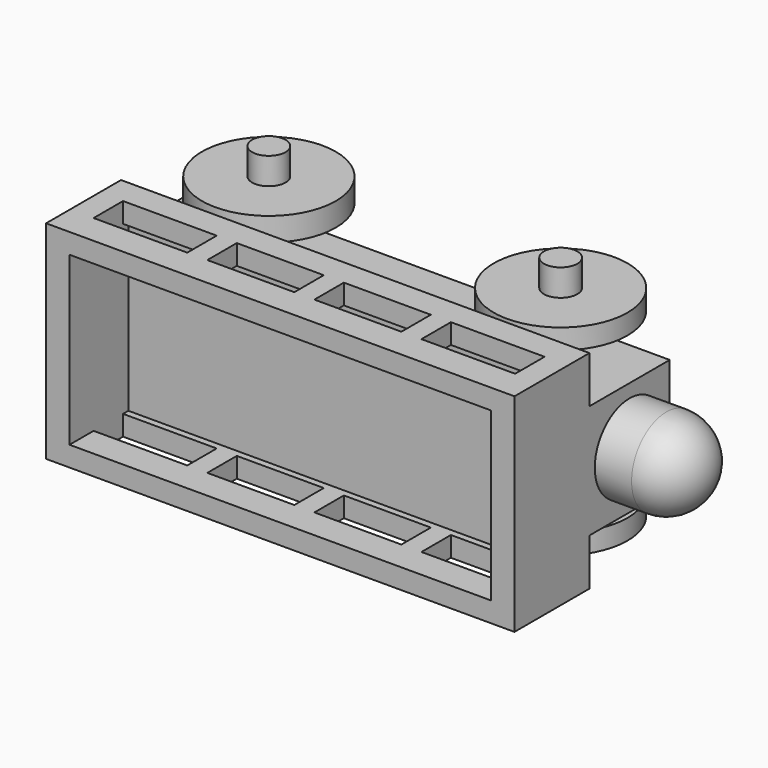
from build123d import *

# Parameters (mm, degrees)
F0_W      = 70
F0_H      = 31
F1_DEPTH  = 1.5
F2_W      = 70
F2_H      = 3
F3_DEPTH  = 11
F4_W      = 70
F4_H      = 3
F5_DEPTH  = 11
F6_W      = 3.5
F6_H      = 25
F7_DEPTH  = 11
F8_W      = 3.5
F8_H      = 25
F9_DEPTH  = 11
F10_W     = 70
F10_H     = 17
F11_DEPTH = 15
F12_W     = 14
F12_H     = 5.5
F13_DEPTH = 70
F14_W     = 13
F14_H     = 5.5
F15_DEPTH = 70
F16_W     = 13
F16_H     = 5.5
F17_DEPTH = 70
F18_W     = 14
F18_H     = 5.5
F19_DEPTH = 70
F21_R     = 3.5
F22_DEPTH = 3.5
F23_R     = 3.5
F24_DEPTH = 3.5
F25_R     = 10
F26_DEPTH = 3
F27_R     = 10
F28_DEPTH = 3.5
F29_R     = 2.5
F30_DEPTH = 4
F31_R     = 2.5
F32_DEPTH = 4
F33_R     = 6.5
F34_DEPTH = 5.5


# Not quite as in the source:
# - a pattern or mirror of a feature is missing from the dataset's text; its kind, count and spacing are read off the source's solid


with BuildPart() as f1:
    # F0 (on Front) → F1 (new body, symmetric)
    with BuildSketch(Plane.XZ):
        Rectangle(F0_W, F0_H)
    extrude(amount=F1_DEPTH, both=True)

    # F2 (on face) → F3 (join)
    with BuildSketch(Plane.XZ.offset(1.5)):
        with Locations((0, -14)):
            Rectangle(F2_W, F2_H)
    extrude(amount=F3_DEPTH)

    # F4 (on face) → F5 (join)
    with BuildSketch(Plane.XZ.offset(1.5)):
        with Locations((0, 14)):
            Rectangle(F4_W, F4_H)
    extrude(amount=F5_DEPTH)

    # F6 (on face) → F7 (join)
    with BuildSketch(Plane.XZ.offset(1.5)):
        with Locations((33.25, 0)):
            Rectangle(F6_W, F6_H)
    extrude(amount=F7_DEPTH)

    # F8 (on face) → F9 (join)
    with BuildSketch(Plane.XZ.offset(1.5)):
        with Locations((-33.25, 0)):
            Rectangle(F8_W, F8_H)
    extrude(amount=F9_DEPTH)

    # F10 (on face) → F11 (join)
    with BuildSketch(Plane(origin=(0, 1.5, 0), x_dir=(-1, 0, 0), z_dir=(0, 1, 0))):
        Rectangle(F10_W, F10_H)
    extrude(amount=F11_DEPTH)

    # F12 (on face) → F13 (cut)
    with BuildSketch(Plane(origin=(0, 0, -15.5), x_dir=(1, 0, 0), z_dir=(0, 0, -1))):
        with Locations((24.5, 5.25)):
            Rectangle(F12_W, F12_H)
    extrude(amount=-F13_DEPTH, mode=Mode.SUBTRACT)

    # F14 (on face) → F15 (cut)
    with BuildSketch(Plane(origin=(0, 0, -15.5), x_dir=(1, 0, 0), z_dir=(0, 0, -1))):
        with Locations((8, 5.25)):
            Rectangle(F14_W, F14_H)
    extrude(amount=-F15_DEPTH, mode=Mode.SUBTRACT)

    # F16 (on face) → F17 (cut)
    with BuildSketch(Plane(origin=(0, 0, -15.5), x_dir=(1, 0, 0), z_dir=(0, 0, -1))):
        with Locations((-8, 5.25)):
            Rectangle(F16_W, F16_H)
    extrude(amount=-F17_DEPTH, mode=Mode.SUBTRACT)

    # F18 (on face) → F19 (cut)
    with BuildSketch(Plane(origin=(0, 0, -15.5), x_dir=(1, 0, 0), z_dir=(0, 0, -1))):
        with Locations((-24.5, 5.25)):
            Rectangle(F18_W, F18_H)
    extrude(amount=-F19_DEPTH, mode=Mode.SUBTRACT)

    # F21 (on face) → F22 (join)
    with BuildSketch(Plane.XY.offset(8.5)):
        with Locations((21.5, 13)):
            Circle(F21_R)
    f22 = extrude(amount=F22_DEPTH)

    # F22_copies: F22 across plane
    add(f22.mirror(Plane(origin=(0, 0, 0), x_dir=(-1, 0, 0), z_dir=(0, 0, -1))))

    # F23 (on face) → F24 (join)
    with BuildSketch(Plane.XY.offset(8.5)):
        with Locations((-22.1062030418, 13)):
            Circle(F23_R)
    f24 = extrude(amount=F24_DEPTH)

    # F24_copies: F24 across plane
    add(f24.mirror(Plane(origin=(0, 0, 0), x_dir=(-1, 0, 0), z_dir=(0, 0, -1))))

    # F25 (on face) → F26 (join)
    with BuildSketch(Plane.XY.offset(12)):
        with Locations((21.5, 13)):
            Circle(F25_R)
    f26 = extrude(amount=F26_DEPTH)

    # F26_copies: F26 across plane
    add(f26.mirror(Plane(origin=(0, 0, 0), x_dir=(-1, 0, 0), z_dir=(0, 0, -1))))

    # F27 (on face) → F28 (join)
    with BuildSketch(Plane.XY.offset(12)):
        with Locations((-22.1062030418, 13)):
            Circle(F27_R)
    f28 = extrude(amount=F28_DEPTH)

    # F28_copies: F28 across plane
    add(f28.mirror(Plane(origin=(0, 0, 0), x_dir=(-1, 0, 0), z_dir=(0, 0, -1))))

    # F29 (on face) → F30 (join)
    with BuildSketch(Plane.XY.offset(15.5)):
        with Locations((-22.1062030418, 13)):
            Circle(F29_R)
    f30 = extrude(amount=F30_DEPTH)

    # F30_copies: F30 across plane
    add(f30.mirror(Plane(origin=(0, 0, 0), x_dir=(-1, 0, 0), z_dir=(0, 0, -1))))

    # F31 (on face) → F32 (join)
    with BuildSketch(Plane.XY.offset(15)):
        with Locations((21.5, 13)):
            Circle(F31_R)
    f32 = extrude(amount=F32_DEPTH)

    # F32_copies: F32 across plane
    add(f32.mirror(Plane(origin=(0, 0, 0), x_dir=(-1, 0, 0), z_dir=(0, 0, -1))))

    # F33 (on face) → F34 (join)
    with BuildSketch(Plane(origin=(-35, 0, 0), x_dir=(0, -1, 0), z_dir=(-1, 0, 0))):
        with Locations((-9, 0)):
            Circle(F33_R)
    f34 = extrude(amount=F34_DEPTH)

    # F34_copies: F34 across plane
    add(f34.mirror(Plane(origin=(0, 0, 0), x_dir=(0, 0, 1), z_dir=(1, 0, 0))))

    # F35 (on face) → F36 (revolve)
    with BuildSketch(Plane(origin=(-40.5, 0, 0), x_dir=(0, -1, 0), z_dir=(-1, 0, 0))):
        with BuildLine():
            Line((-15.5, 0), (-9, 0))
            Line((-9, 0), (-2.5, 0))
            ThreePointArc((-2.5, 0), (-9, 6.5), (-15.5, 0))
        make_face()
    f36 = revolve(axis=Axis((-40.5, 9, 0), (0, 1, 0)))

    # F36_copies: F36 across plane
    add(f36.mirror(Plane(origin=(0, 0, 0), x_dir=(0, 0, 1), z_dir=(1, 0, 0))))


solid = f1.part
